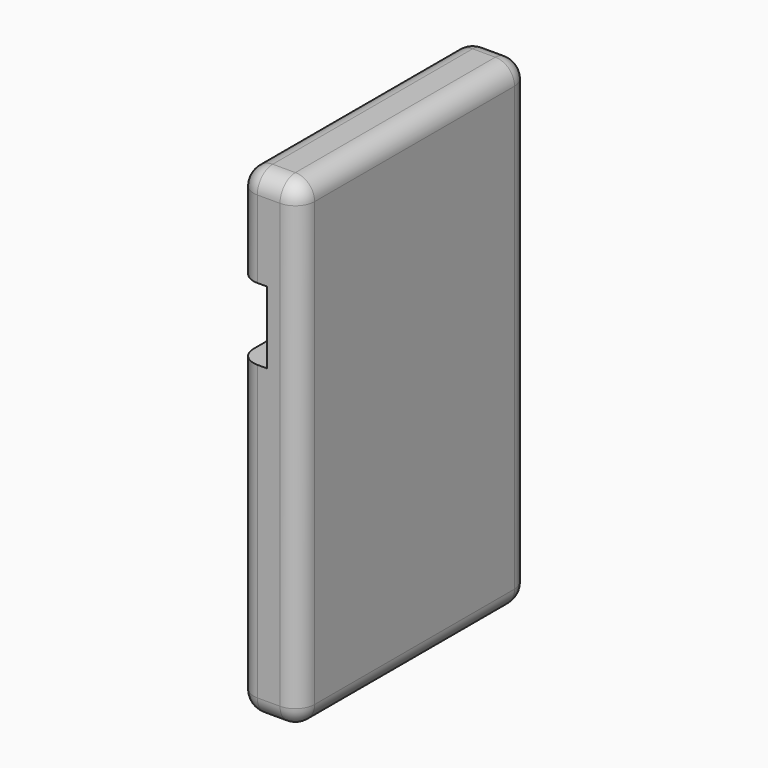
from build123d import *

# Parameters (mm, degrees)
F1_DEPTH     = 76.2
F2_R         = 5.08
F3_R         = 5.08
F4_T1_DEPTH  = 5.998990562
F4_S5_W      = 5.08
F4_S5_H      = 5.08
F4_T6_DEPTH  = 5.08
F4_S11_W     = 5.08
F4_S11_H     = 5.08
F4_T12_DEPTH = 5.08
F4_S17_W     = 5.08
F4_S17_H     = 5.08
F4_T18_DEPTH = 5.08
F4_S23_W     = 5.08
F4_S23_H     = 5.08
F4_T24_DEPTH = 5.08
F4_S29_W     = 5.08
F4_S29_H     = 5.08
F4_T30_DEPTH = 5.08
F4_S35_W     = 5.08
F4_S35_H     = 5.08
F4_T36_DEPTH = 5.08


# Not quite as in the source:
# - a fillet or chamfer that OpenCascade refuses, or shapes differently, is made with other operations: its cross-section is extruded or revolved along the edge and cut away or added


with BuildPart() as f1:
    # F0 (on Front) → F1 (new body)
    with BuildSketch(Plane.XZ):
        Polygon((-16.158990562, 0), (0, 0), (0, 127.1478682756), (-16.158990562, 127.1478682756), (-16.158990562, 101.6), (-8.5426843725, 101.6), (-8.5426843725, 82.55), (-16.158990562, 82.55), align=None)
    extrude(amount=F1_DEPTH)

    # F2
    f2_edges = [f1.edges().sort_by_distance(p)[0] for p in [
        (-8.079495, -76.2, 127.147868),
        (0, -38.1, 0),
        (0, -38.1, 127.147868),
        (0, 0, 63.573934),
        (0, -76.2, 63.573934),
    ]]
    fillet(f2_edges, radius=F2_R)

    # F3
    f3_edges = [f1.edges().sort_by_distance(p)[0] for p in [
        (-16.158991, -76.2, 41.275),
        (-16.158991, 0, 41.275),
        (-16.158991, -38.1, 0),
        (-16.158991, 0, 114.373934),
        (-16.158991, -35.56, 127.147868),
    ]]
    fillet(f3_edges, radius=F3_R)

    # F4: fillet of radius 5.08 on 3 edges, made by hand

    # F4_s2 → F4_t1 (cut)
    with BuildSketch(Plane.YZ.offset(-11.078990562)):
        with BuildLine():
            ThreePointArc((0, 122.0678682756), (-1.4878975516, 125.6599707241), (-5.08, 127.1478682756))
            Line((-5.08, 127.1478682756), (0, 127.1478682756))
            Line((0, 127.1478682756), (0, 122.0678682756))
        make_face()
        with BuildLine():
            ThreePointArc((-5.08, 0), (-1.4878975516, 1.4878975516), (0, 5.08))
            Line((0, 5.08), (0, 0))
            Line((0, 0), (-5.08, 0))
        make_face()
        with BuildLine():
            ThreePointArc((-71.12, 0), (-74.7121024484, 1.4878975516), (-76.2, 5.08))
            Line((-76.2, 5.08), (-76.2, 0))
            Line((-76.2, 0), (-71.12, 0))
        make_face()
    extrude(amount=F4_T1_DEPTH, mode=Mode.SUBTRACT)


with BuildPart() as f4_tool4:
    # F4_s5 → F4_t6 (new body)
    with BuildSketch(Plane.XY.offset(5.08)):
        with Locations((-13.618990562, -73.66)):
            Rectangle(F4_S5_W, F4_S5_H)
    extrude(amount=-F4_T6_DEPTH)

    # F4_s7 → F4_t8 (revolve, cut)
    with BuildSketch(Plane(origin=(-11.078990562, -71.12, 5.08), x_dir=(0.7071067812, 0.7071067812, 0), z_dir=(-0.7071067812, 0.7071067812, 0))):
        with BuildLine():
            ThreePointArc((0, -5.08), (5.08, 0), (0, 5.08))
            Line((0, 5.08), (0, -5.08))
        make_face()
    revolve(axis=Axis((-11.078990562, -71.12, 5.08), (0, 0, -1)), mode=Mode.SUBTRACT)


with BuildPart() as f1_1:
    add(f1.part)

    # F4_t3: cut F4_tool4
    add(f4_tool4.part, mode=Mode.SUBTRACT)


with BuildPart() as f4_tool10:
    # F4_s11 → F4_t12 (new body)
    with BuildSketch(Plane.XY.offset(5.08)):
        with Locations((-2.54, -73.66)):
            Rectangle(F4_S11_W, F4_S11_H)
    extrude(amount=-F4_T12_DEPTH)

    # F4_s13 → F4_t14 (revolve, cut)
    with BuildSketch(Plane(origin=(-5.08, -71.12, 5.08), x_dir=(-0.7071067812, 0.7071067812, 0), z_dir=(-0.7071067812, -0.7071067812, 0))):
        with BuildLine():
            ThreePointArc((0, -5.08), (5.08, 0), (0, 5.08))
            Line((0, 5.08), (0, -5.08))
        make_face()
    revolve(axis=Axis((-5.08, -71.12, 5.08), (0, 0, -1)), mode=Mode.SUBTRACT)


with BuildPart() as f1_2:
    add(f1_1.part)

    # F4_t9: cut F4_tool10
    add(f4_tool10.part, mode=Mode.SUBTRACT)


with BuildPart() as f4_tool16:
    # F4_s17 → F4_t18 (new body)
    with BuildSketch(Plane.XY.offset(5.08)):
        with Locations((-13.618990562, -2.54)):
            Rectangle(F4_S17_W, F4_S17_H)
    extrude(amount=-F4_T18_DEPTH)

    # F4_s19 → F4_t20 (revolve, cut)
    with BuildSketch(Plane(origin=(-11.078990562, -5.08, 5.08), x_dir=(0.7071067812, -0.7071067812, 0), z_dir=(0.7071067812, 0.7071067812, 0))):
        with BuildLine():
            ThreePointArc((0, -5.08), (5.08, 0), (0, 5.08))
            Line((0, 5.08), (0, -5.08))
        make_face()
    revolve(axis=Axis((-11.078990562, -5.08, 5.08), (0, 0, -1)), mode=Mode.SUBTRACT)


with BuildPart() as f1_3:
    add(f1_2.part)

    # F4_t15: cut F4_tool16
    add(f4_tool16.part, mode=Mode.SUBTRACT)


with BuildPart() as f4_tool22:
    # F4_s23 → F4_t24 (new body)
    with BuildSketch(Plane.XY.offset(5.08)):
        with Locations((-2.54, -2.54)):
            Rectangle(F4_S23_W, F4_S23_H)
    extrude(amount=-F4_T24_DEPTH)

    # F4_s25 → F4_t26 (revolve, cut)
    with BuildSketch(Plane(origin=(-5.08, -5.08, 5.08), x_dir=(-0.7071067812, -0.7071067812, 0), z_dir=(0.7071067812, -0.7071067812, 0))):
        with BuildLine():
            ThreePointArc((0, -5.08), (5.08, 0), (0, 5.08))
            Line((0, 5.08), (0, -5.08))
        make_face()
    revolve(axis=Axis((-5.08, -5.08, 5.08), (0, 0, -1)), mode=Mode.SUBTRACT)


with BuildPart() as f1_4:
    add(f1_3.part)

    # F4_t21: cut F4_tool22
    add(f4_tool22.part, mode=Mode.SUBTRACT)


with BuildPart() as f4_tool28:
    # F4_s29 → F4_t30 (new body)
    with BuildSketch(Plane.XZ.offset(5.08)):
        with Locations((-2.54, 124.6078682756)):
            Rectangle(F4_S29_W, F4_S29_H)
    extrude(amount=-F4_T30_DEPTH)

    # F4_s31 → F4_t32 (revolve, cut)
    with BuildSketch(Plane(origin=(-5.08, -5.08, 122.0678682756), x_dir=(-0.7071067812, 0, -0.7071067812), z_dir=(0.7071067812, 0, -0.7071067812))):
        with BuildLine():
            ThreePointArc((0, -5.08), (5.08, 0), (0, 5.08))
            Line((0, 5.08), (0, -5.08))
        make_face()
    revolve(axis=Axis((-5.08, -5.08, 122.0678682756), (0, 1, 0)), mode=Mode.SUBTRACT)


with BuildPart() as f1_5:
    add(f1_4.part)

    # F4_t27: cut F4_tool28
    add(f4_tool28.part, mode=Mode.SUBTRACT)


with BuildPart() as f4_tool34:
    # F4_s35 → F4_t36 (new body)
    with BuildSketch(Plane.XZ.offset(5.08)):
        with Locations((-13.618990562, 124.6078682756)):
            Rectangle(F4_S35_W, F4_S35_H)
    extrude(amount=-F4_T36_DEPTH)

    # F4_s37 → F4_t38 (revolve, cut)
    with BuildSketch(Plane(origin=(-11.078990562, -5.08, 122.0678682756), x_dir=(0.7071067812, 0, -0.7071067812), z_dir=(0.7071067812, 0, 0.7071067812))):
        with BuildLine():
            ThreePointArc((0, -5.08), (5.08, 0), (0, 5.08))
            Line((0, 5.08), (0, -5.08))
        make_face()
    revolve(axis=Axis((-11.078990562, -5.08, 122.0678682756), (0, 1, 0)), mode=Mode.SUBTRACT)


with BuildPart() as f1_6:
    add(f1_5.part)

    # F4_t33: cut F4_tool34
    add(f4_tool34.part, mode=Mode.SUBTRACT)


solid = f1_6.part
